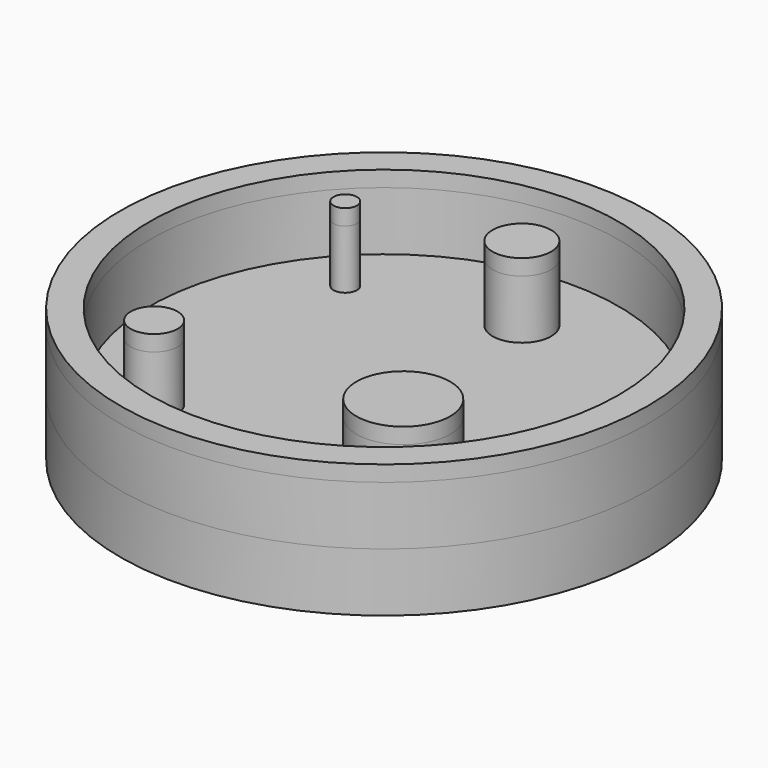
from build123d import *

# Parameters (mm, degrees)
F0_R        = 22.5
F0_R_2      = 20
F1_DEPTH    = 5
F0_R_3      = 4
F0_R_4      = 2.5
F0_R_5      = 1
F0_R_6      = 2
F1_FACE_R   = 22.5
F1_FACE_R_2 = 20
F2_DEPTH    = 5
F5_DEPTH    = 5
F6_DEPTH    = 1.35


# Not quite as in the source:
# - a feature of the source that left no trace in its solid (it failed there, or was rolled back) is left out
# - the program builds the solid bodies; features that only make, move or delete a surface that nothing else refers to are left out


with BuildPart() as f1:
    # F0 (on Top) → F1 (new body)
    with BuildSketch(Plane.XY):
        with Locations((-20.9074081164, 13.653905517)):
            Circle(F0_R)
        with Locations((-20.9074081164, 13.653905517)):
            Circle(F0_R_2, mode=Mode.SUBTRACT)
    extrude(amount=F1_DEPTH)

    # F1_face (on face) + F0 (on Top) → F2 (join)
    with BuildSketch(Plane(origin=(-20.9074081164, 13.653905517, 5), x_dir=(1, 0, 0), z_dir=(0, 0, 1))):
        Circle(F1_FACE_R)
        Circle(F1_FACE_R_2, mode=Mode.SUBTRACT)
    with BuildSketch(Plane.XY):
        with Locations((-20.9074081164, 13.653905517)):
            Circle(F0_R)
        with Locations((-20.9074081164, 13.653905517)):
            Circle(F0_R_2, mode=Mode.SUBTRACT)
        with Locations((-20.9074081164, 13.653905517)):
            Circle(F0_R_2)
        with Locations((-31.7896045744, 2.7569008525)):
            Circle(F0_R_6, mode=Mode.SUBTRACT)
        with Locations((-11.7507977411, 4.2523336597)):
            Circle(F0_R_3, mode=Mode.SUBTRACT)
        with Locations((-32.5716212392, 24.0953601897)):
            Circle(F0_R_5, mode=Mode.SUBTRACT)
        with Locations((-19.8261346668, 26.982922107)):
            Circle(F0_R_4, mode=Mode.SUBTRACT)
    extrude(amount=-F2_DEPTH)


with BuildPart() as f1b:
    # F0 (on Top) → F1, piece 2 (new body)
    with BuildSketch(Plane.XY):
        with Locations((-11.7507977411, 4.2523336597)):
            Circle(F0_R_3)
    extrude(amount=F1_DEPTH)


with BuildPart() as f1c:
    # F0 (on Top) → F1, piece 3 (new body)
    with BuildSketch(Plane.XY):
        with Locations((-19.8261346668, 26.982922107)):
            Circle(F0_R_4)
    extrude(amount=F1_DEPTH)


with BuildPart() as f1d:
    # F0 (on Top) → F1, piece 4 (new body)
    with BuildSketch(Plane.XY):
        with Locations((-32.5716212392, 24.0953601897)):
            Circle(F0_R_5)
    extrude(amount=F1_DEPTH)


with BuildPart() as f1e:
    # F0 (on Top) → F1, piece 5 (new body)
    with BuildSketch(Plane.XY):
        with Locations((-31.7896045744, 2.7569008525)):
            Circle(F0_R_6)
    extrude(amount=F1_DEPTH)


with BuildPart() as f5:
    # F0 (on Top) → F5 (new body)
    with BuildSketch(Plane.XY):
        with Locations((-11.7507977411, 4.2523336597)):
            Circle(F0_R_3)
    extrude(amount=-F5_DEPTH)


with BuildPart() as f5b:
    # F0 (on Top) → F5, piece 2 (new body)
    with BuildSketch(Plane.XY):
        with Locations((-31.7896045744, 2.7569008525)):
            Circle(F0_R_6)
    extrude(amount=-F5_DEPTH)


with BuildPart() as f5c:
    # F0 (on Top) → F5, piece 3 (new body)
    with BuildSketch(Plane.XY):
        with Locations((-32.5716212392, 24.0953601897)):
            Circle(F0_R_5)
    extrude(amount=-F5_DEPTH)


with BuildPart() as f5d:
    # F0 (on Top) → F5, piece 4 (new body)
    with BuildSketch(Plane.XY):
        with Locations((-19.8261346668, 26.982922107)):
            Circle(F0_R_4)
    extrude(amount=-F5_DEPTH)


with BuildPart() as f6:
    # F6 (new): a face of the model
    f6_faces = [f1.part.faces().sort_by_distance(p)[0] for p in [
        (-42.7710120133, 13.653905517, 5),
    ]]
    extrude(f6_faces, amount=F6_DEPTH)


with BuildPart() as f6b:
    # F6#2 (new): a face of the model
    f6_2_faces = [f1e.part.faces().sort_by_distance(p)[0] for p in [
        (-31.7896045744, 2.7569008525, 5),
    ]]
    extrude(f6_2_faces, amount=F6_DEPTH)


with BuildPart() as f6c:
    # F6#3 (new): a face of the model
    f6_3_faces = [f1d.part.faces().sort_by_distance(p)[0] for p in [
        (-32.5716212392, 24.0953601897, 5),
    ]]
    extrude(f6_3_faces, amount=F6_DEPTH)


with BuildPart() as f6d:
    # F6#4 (new): a face of the model
    f6_4_faces = [f1b.part.faces().sort_by_distance(p)[0] for p in [
        (-11.7507977411, 4.2523336597, 5),
    ]]
    extrude(f6_4_faces, amount=F6_DEPTH)


with BuildPart() as f6e:
    # F6#5 (new): a face of the model
    f6_5_faces = [f1c.part.faces().sort_by_distance(p)[0] for p in [
        (-19.8261346668, 26.982922107, 5),
    ]]
    extrude(f6_5_faces, amount=F6_DEPTH)


solid = Compound([f1.part, f1b.part, f1c.part, f1d.part, f1e.part, f5.part, f5b.part, f5c.part, f5d.part, f6.part, f6b.part, f6c.part, f6d.part, f6e.part])
